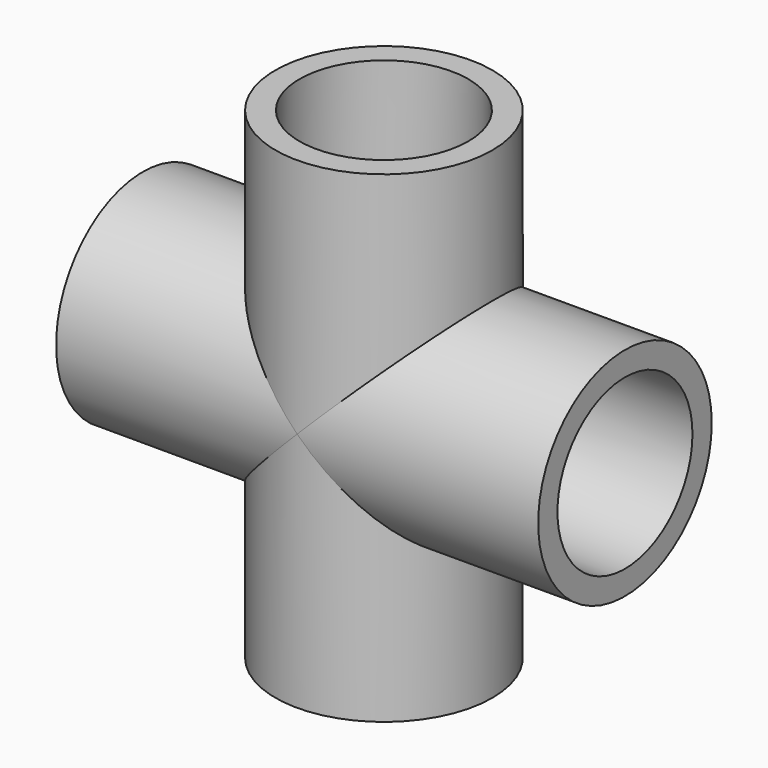
from build123d import *
from build123d import SkipClean  # not in build123d's __all__

# Parameters (mm, degrees)
F0_R     = 14.2875
F0_R_2   = 11.1125
F1_DEPTH = 31.75
F0_R_3   = 10.31875
F2_DEPTH = 14.2875
F3_R     = 14.2875
F3_R_2   = 11.1125
F4_DEPTH = 31.75
F3_R_3   = 10.31875
F5_DEPTH = 14.2875
F6_DEPTH = 14.2875
F7_DEPTH = 14.2875


with BuildPart() as f1:
    # F0 (on Top) → F1 (new body, symmetric)
    with BuildSketch(Plane.XY):
        Circle(F0_R)
        Circle(F0_R_2, mode=Mode.SUBTRACT)
    extrude(amount=F1_DEPTH, both=True)

    # F0 (on Top) → F2 (join, symmetric)
    with BuildSketch(Plane.XY):
        Circle(F0_R_2)
        Circle(F0_R_3, mode=Mode.SUBTRACT)
    extrude(amount=F2_DEPTH, both=True)

    # F3 (on Right) → F4 (join, symmetric)
    with BuildSketch(Plane.YZ):
        Circle(F3_R)
        Circle(F3_R_2, mode=Mode.SUBTRACT)
    extrude(amount=F4_DEPTH, both=True)

    # F3 (on Right) → F5 (join, symmetric)
    with BuildSketch(Plane.YZ):
        Circle(F3_R_2)
        Circle(F3_R_3, mode=Mode.SUBTRACT)
    with SkipClean():  # cleaning this boolean's faces spoils the solid; the shape is the same uncleaned
        extrude(amount=F5_DEPTH, both=True)

    # F0 (on Top) → F6 (cut, symmetric)
    with BuildSketch(Plane.XY):
        Circle(F0_R_3)
    with SkipClean():  # cleaning this boolean's faces spoils the solid; the shape is the same uncleaned
        extrude(amount=F6_DEPTH, both=True, mode=Mode.SUBTRACT)

    # F3 (on Right) → F7 (cut, symmetric)
    with BuildSketch(Plane.YZ):
        Circle(F3_R_3)
    extrude(amount=F7_DEPTH, both=True, mode=Mode.SUBTRACT)


solid = f1.part
